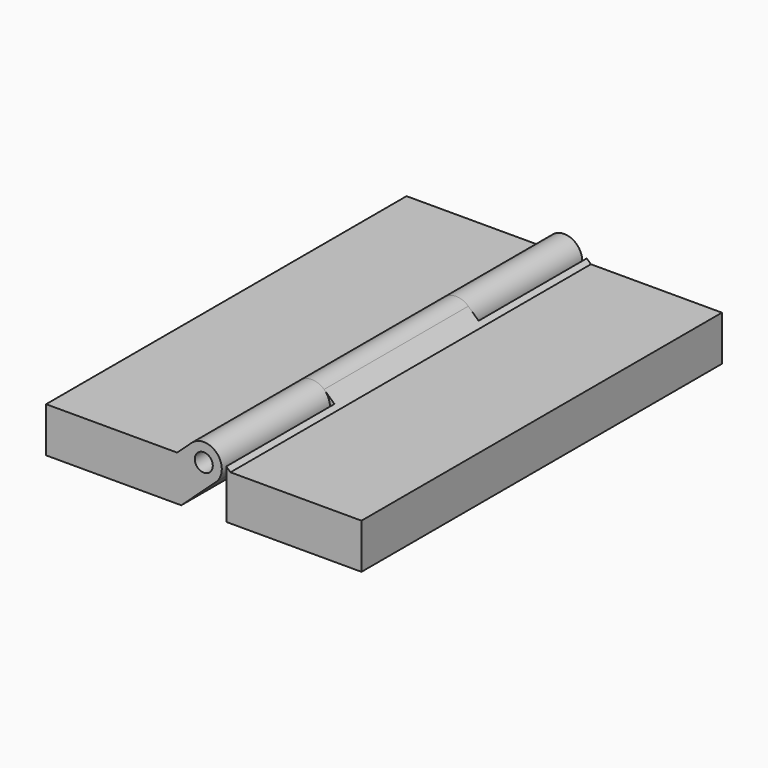
from build123d import *

# Parameters (mm, degrees)
F0_R     = 0.254
F1_DEPTH = 6.35
F2_R     = 0.254
F3_DEPTH = 6.35
F4_W     = 1.27
F4_H     = 5.08
F5_DEPTH = 1.779
F4_H_2   = 6.35
F6_DEPTH = 1.779


with BuildPart() as f1:
    # F0 (on Front) → F1 (new body, symmetric)
    with BuildSketch(Plane.XZ):
        with BuildLine():
            Line((-0.9780140565, 0.8952929717), (0, 0))
            Line((0, 0), (3.81, 0))
            Line((3.81, 0), (3.81, 1.27))
            Line((3.81, 1.27), (0.117342346, 1.27))
            Line((0.117342346, 1.27), (-0.2919859435, 1.6447070283))
            ThreePointArc((-0.2919859435, 1.6447070283), (-0.1700725106, 1.4747105997), (-0.127, 1.27))
            ThreePointArc((-0.127, 1.27), (-0.4302894003, 0.8050725106), (-0.9780140565, 0.8952929717))
        make_face()
        with BuildLine():
            ThreePointArc((-0.2919859435, 1.6447070283), (-1.0097070283, 1.6130140565), (-0.9780140565, 0.8952929717))
            ThreePointArc((-0.9780140565, 0.8952929717), (-0.4302894003, 0.8050725106), (-0.127, 1.27))
            ThreePointArc((-0.127, 1.27), (-0.1700725106, 1.4747105997), (-0.2919859435, 1.6447070283))
        make_face()
        with Locations((-0.635, 1.27)):
            Circle(F0_R, mode=Mode.SUBTRACT)
    extrude(amount=F1_DEPTH, both=True)

    # F4 (on Top) → F6 (cut, through all)
    with BuildSketch(Plane.XY):
        with Locations((-0.635, 5.715)):
            Rectangle(F4_W, F4_H_2)
        with Locations((-0.635, -5.715)):
            Rectangle(F4_W, F4_H_2)
    extrude(amount=F6_DEPTH, mode=Mode.SUBTRACT)


with BuildPart() as f3:
    # F2 (on Front) → F3 (new body, symmetric)
    with BuildSketch(Plane.XZ):
        with BuildLine():
            Line((-1.27, 0), (-0.2919859435, 0.8952929717))
            ThreePointArc((-0.2919859435, 0.8952929717), (-0.2602929717, 1.6130140565), (-0.9780140565, 1.6447070283))
            Line((-0.9780140565, 1.6447070283), (-1.387342346, 1.27))
            Line((-1.387342346, 1.27), (-5.08, 1.27))
            Line((-5.08, 1.27), (-5.08, 0))
            Line((-5.08, 0), (-1.27, 0))
        make_face()
        with Locations((-0.635, 1.27)):
            Circle(F2_R, mode=Mode.SUBTRACT)
    extrude(amount=F3_DEPTH, both=True)

    # F4 (on Top) → F5 (cut, through all)
    with BuildSketch(Plane.XY):
        with Locations((-0.635, 0)):
            Rectangle(F4_W, F4_H)
    extrude(amount=F5_DEPTH, mode=Mode.SUBTRACT)


solid = Compound([f1.part, f3.part])
